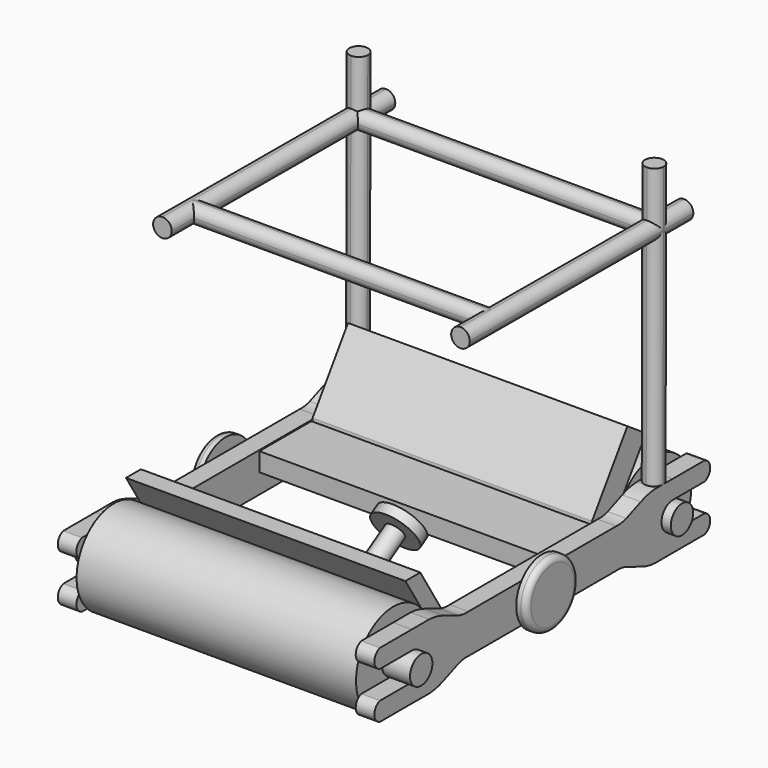
from build123d import *

# Parameters (mm, degrees)
F0_R           = 5
F1_DEPTH       = 30
F2_R           = 1.5
F3_DEPTH       = 3
F3_DEPTH_BACK  = 33
F5_DEPTH       = 2
F7_DEPTH       = 2
F8_R           = 3.5
F9_DEPTH       = 1.1
F10_R          = 0.6
F11_W          = 2
F11_H          = 2
F12_DEPTH      = 30
F13_W          = 2
F13_H          = 2
F14_DEPTH      = 25
F14_DEPTH_BACK = 5
F15_W          = 2
F15_H          = 1.9935706709
F16_DEPTH      = 31
F16_DEPTH_BACK = 1
F18_DEPTH      = 30
F19_R          = 1
F20_DEPTH      = 4.6
F21_R          = 2.5
F22_DEPTH      = 1.1
F23_R          = 0.99999
F24_R          = 0.99999
F25_R          = 0.99999
F26_R          = 0.99999
F27_T1_DEPTH   = 37
F28_T1_DEPTH   = 37
F29_R          = 3.5
F30_DEPTH      = 1.1
F31_R          = 0.6


# Not quite as in the source:
# - a fillet or chamfer that OpenCascade refuses, or shapes differently, is made with other operations: its cross-section is extruded or revolved along the edge and cut away or added
# - a fillet or chamfer is up to 0.001 mm smaller than in the source, because OpenCascade refuses the exact size


with BuildPart() as f1:
    # F0 (on Right) → F1 (new body)
    with BuildSketch(Plane.YZ):
        Circle(F0_R)
        with Locations((-35, 0)):
            Circle(F0_R)
    extrude(amount=F1_DEPTH)

    # F2 (on face) → F3 (join, two sides)
    with BuildSketch(Plane.YZ.offset(30)) as f3_sk:
        Circle(F2_R)
        with Locations((-35, 0)):
            Circle(F2_R)
    extrude(amount=F3_DEPTH)
    extrude(f3_sk.sketch, amount=-F3_DEPTH_BACK)


with BuildPart() as f5:
    # F4 (on face) → F5 (new body)
    with BuildSketch(Plane.YZ.offset(30)):
        with BuildLine():
            Line((-32.6922312379, 3.5074306652), (-35, 3.5))
            Line((-35, 3.5), (-39.2814344682, 3.5))
            ThreePointArc((-39.2814344682, 3.5), (-40.0388480928, 2.5), (-39.2814344682, 1.5))
            Line((-39.2814344682, 1.5), (-35, 1.5))
            ThreePointArc((-35, 1.5), (-33.9393398282, 1.0606601718), (-33.5, 0))
            ThreePointArc((-33.5, 0), (-33.9393398282, -1.0606601718), (-35, -1.5))
            Line((-35, -1.5), (-39.2814344682, -1.5))
            ThreePointArc((-39.2814344682, -1.5), (-40.0388480928, -2.5), (-39.2814344682, -3.5))
            Line((-39.2814344682, -3.5), (-35, -3.5))
            Line((-35, -3.5), (-32.6922312379, -3.5074306652))
            ThreePointArc((-32.6922312379, -3.5074306652), (-31.6914030649, -3.3770056429), (-30.7308007418, -3.0673108011))
            Line((-30.7308007418, -3.0673108011), (-28.7733972073, -2.2878439631))
            ThreePointArc((-28.7733972073, -2.2878439631), (-28.1066667518, -2.1263179414), (-27.4209757003, -2.1051533986))
            Line((-27.4209757003, -2.1051533986), (-17.5, -2.1051533986))
            Line((-17.5, -2.1051533986), (-7.5790242997, -2.1051533986))
            ThreePointArc((-7.5790242997, -2.1051533986), (-6.8933332482, -2.1263179414), (-6.2266027927, -2.2878439631))
            Line((-6.2266027927, -2.2878439631), (-4.2691992582, -3.0673108011))
            ThreePointArc((-4.2691992582, -3.0673108011), (-3.3085969351, -3.3770056429), (-2.3077687621, -3.5074306652))
            Line((-2.3077687621, -3.5074306652), (0, -3.5))
            Line((0, -3.5), (4.2814344682, -3.5))
            ThreePointArc((4.2814344682, -3.5), (5.0388480928, -2.5), (4.2814344682, -1.5))
            Line((4.2814344682, -1.5), (0, -1.5))
            ThreePointArc((0, -1.5), (-1.0606601718, -1.0606601718), (-1.5, 0))
            ThreePointArc((-1.5, 0), (-1.0606601718, 1.0606601718), (0, 1.5))
            Line((0, 1.5), (4.2814344682, 1.5))
            ThreePointArc((4.2814344682, 1.5), (5.0388480928, 2.5), (4.2814344682, 3.5))
            Line((4.2814344682, 3.5), (0, 3.5))
            Line((0, 3.5), (-2.3077687621, 3.5074306652))
            ThreePointArc((-2.3077687621, 3.5074306652), (-3.3085969351, 3.3770056429), (-4.2691992582, 3.0673108011))
            Line((-4.2691992582, 3.0673108011), (-6.2266027927, 2.2878439631))
            ThreePointArc((-6.2266027927, 2.2878439631), (-6.8933332482, 2.1263179414), (-7.5790242997, 2.1051533986))
            Line((-7.5790242997, 2.1051533986), (-17.5, 2.1051533986))
            Line((-17.5, 2.1051533986), (-27.4209757003, 2.1051533986))
            ThreePointArc((-27.4209757003, 2.1051533986), (-28.1066667518, 2.1263179414), (-28.7733972073, 2.2878439631))
            Line((-28.7733972073, 2.2878439631), (-30.7308007418, 3.0673108011))
            ThreePointArc((-30.7308007418, 3.0673108011), (-31.6914030649, 3.3770056429), (-32.6922312379, 3.5074306652))
        make_face()
    extrude(amount=F5_DEPTH)

    # F8 (on face) → F9 (join)
    with BuildSketch(Plane.YZ.offset(32)):
        with Locations((-17.5, 0)):
            Circle(F8_R)
    extrude(amount=F9_DEPTH)

    # F10
    f10_edges = [f5.edges().sort_by_distance(p)[0] for p in [
        (33.1, -21, 0),
    ]]
    fillet(f10_edges, radius=F10_R)


with BuildPart() as f7:
    # F6 (on face) → F7 (new body)
    with BuildSketch(Plane(origin=(0, 0, 0), x_dir=(0, -1, 0), z_dir=(-1, 0, 0))):
        with BuildLine():
            Line((2.2948030382, 3.5074306652), (-0.0129657239, 3.5))
            Line((-0.0129657239, 3.5), (-4.2944001921, 3.5))
            ThreePointArc((-4.2944001921, 3.5), (-5.0518138167, 2.5), (-4.2944001921, 1.5))
            Line((-4.2944001921, 1.5), (-0.0129657239, 1.5))
            ThreePointArc((-0.0129657239, 1.5), (1.0476944479, 1.0606601718), (1.4870342761, 0))
            ThreePointArc((1.4870342761, 0), (1.0476944479, -1.0606601718), (-0.0129657239, -1.5))
            Line((-0.0129657239, -1.5), (-4.2944001921, -1.5))
            ThreePointArc((-4.2944001921, -1.5), (-5.0518138167, -2.5), (-4.2944001921, -3.5))
            Line((-4.2944001921, -3.5), (-0.0129657239, -3.5))
            Line((-0.0129657239, -3.5), (2.2948030382, -3.5074306652))
            ThreePointArc((2.2948030382, -3.5074306652), (3.2956312112, -3.3770056429), (4.2562335343, -3.0673108011))
            Line((4.2562335343, -3.0673108011), (6.2136370689, -2.2878439631))
            ThreePointArc((6.2136370689, -2.2878439631), (6.8803675243, -2.1263179414), (7.5660585758, -2.1051533986))
            Line((7.5660585758, -2.1051533986), (17.4870342761, -2.1051533986))
            Line((17.4870342761, -2.1051533986), (27.4080099764, -2.1051533986))
            ThreePointArc((27.4080099764, -2.1051533986), (28.0937010279, -2.1263179414), (28.7604314834, -2.2878439631))
            Line((28.7604314834, -2.2878439631), (30.7178350179, -3.0673108011))
            ThreePointArc((30.7178350179, -3.0673108011), (31.6784373411, -3.3770056429), (32.679265514, -3.5074306652))
            Line((32.679265514, -3.5074306652), (34.9870342761, -3.5))
            Line((34.9870342761, -3.5), (39.2684687444, -3.5))
            ThreePointArc((39.2684687444, -3.5), (40.0258823689, -2.5), (39.2684687444, -1.5))
            Line((39.2684687444, -1.5), (34.9870342761, -1.5))
            ThreePointArc((34.9870342761, -1.5), (33.9263741043, -1.0606601718), (33.4870342761, 0))
            ThreePointArc((33.4870342761, 0), (33.9263741043, 1.0606601718), (34.9870342761, 1.5))
            Line((34.9870342761, 1.5), (39.2684687444, 1.5))
            ThreePointArc((39.2684687444, 1.5), (40.0258823689, 2.5), (39.2684687444, 3.5))
            Line((39.2684687444, 3.5), (34.9870342761, 3.5))
            Line((34.9870342761, 3.5), (32.679265514, 3.5074306652))
            ThreePointArc((32.679265514, 3.5074306652), (31.6784373411, 3.3770056429), (30.7178350179, 3.0673108011))
            Line((30.7178350179, 3.0673108011), (28.7604314834, 2.2878439631))
            ThreePointArc((28.7604314834, 2.2878439631), (28.0937010279, 2.1263179414), (27.4080099764, 2.1051533986))
            Line((27.4080099764, 2.1051533986), (17.4870342761, 2.1051533986))
            Line((17.4870342761, 2.1051533986), (7.5660585758, 2.1051533986))
            ThreePointArc((7.5660585758, 2.1051533986), (6.8803675243, 2.1263179414), (6.2136370689, 2.2878439631))
            Line((6.2136370689, 2.2878439631), (4.2562335343, 3.0673108011))
            ThreePointArc((4.2562335343, 3.0673108011), (3.2956312112, 3.3770056429), (2.2948030382, 3.5074306652))
        make_face()
    extrude(amount=F7_DEPTH)

    # F29 (on face) → F30 (join)
    with BuildSketch(Plane(origin=(-2, 0, 0), x_dir=(0, -1, 0), z_dir=(-1, 0, 0))):
        with Locations((17.5, 0)):
            Circle(F29_R)
    extrude(amount=F30_DEPTH)

    # F31
    f31_edges = [f7.edges().sort_by_distance(p)[0] for p in [
        (-3.1, -14, 0),
    ]]
    fillet(f31_edges, radius=F31_R)


with BuildPart() as f12:
    # F11 (on face) → F12 (new body)
    with BuildSketch(Plane(origin=(0, 0.011269352, 3.4999637144), x_dir=(1, 0, 0), z_dir=(0, 0.0032198316, 0.9999948163))):
        with Locations((31, -1.3190501353)):
            Rectangle(F11_W, F11_H)
        Polygon((-2.042085199, -1.9569919301), (-0.0425376123, -1.9995295424), (0, 1.80443e-05), (-1.9995475867, 0.0425556566), align=None)
    extrude(amount=F12_DEPTH)

    # F23 (radius 1 in the source; OpenCascade refuses exactly that, so slightly less here)
    f23_edges = [f12.edges().sort_by_distance(p)[0] for p in [
        (-2.042085, -1.897415, 18.506187),
        (-1.999548, 0.102122, 18.499749),
        (-0.042538, -1.939952, 18.506324),
        (0, 0.059585, 18.499886),
    ]]
    fillet(f23_edges, radius=F23_R)

    # F24 (radius 1 in the source; OpenCascade refuses exactly that, so slightly less here)
    f24_edges = [f12.edges().sort_by_distance(p)[0] for p in [
        (30, -0.259482, 18.500913),
        (32, -2.259471, 18.507353),
        (32, -0.259482, 18.500913),
        (30, -2.259471, 18.507353),
    ]]
    fillet(f24_edges, radius=F24_R)


with BuildPart() as f14:
    # F13 (on face) → F14 (new body, two sides)
    with BuildSketch(Plane(origin=(0, -2.3190381141, 0.0074669508), x_dir=(1, 0, 0), z_dir=(0, -0.9999948163, 0.0032198316))) as f14_sk:
        with Locations((31, 27.4999818572)):
            Rectangle(F13_W, F13_H)
        with Locations((-1, 27.4999818572)):
            Rectangle(F13_W, F13_H)
    extrude(amount=F14_DEPTH)
    extrude(f14_sk.sketch, amount=-F14_DEPTH_BACK)

    # F25 (radius 1 in the source; OpenCascade refuses exactly that, so slightly less here)
    f25_edges = [f14.edges().sort_by_distance(p)[0] for p in [
        (32, -12.227221, 28.539499),
        (32, -12.233661, 26.53951),
        (30, -12.227221, 28.539499),
        (30, -12.233661, 26.53951),
    ]]
    fillet(f25_edges, radius=F25_R)

    # F26 (radius 1 in the source; OpenCascade refuses exactly that, so slightly less here)
    f26_edges = [f14.edges().sort_by_distance(p)[0] for p in [
        (-2, -12.227221, 28.539499),
        (0, -12.227221, 28.539499),
        (-2, -12.233661, 26.53951),
        (0, -12.233661, 26.53951),
    ]]
    fillet(f26_edges, radius=F26_R)


with BuildPart() as f16:
    # F15 (on face) → F16 (new body, two sides)
    with BuildSketch(Plane(origin=(30, 0, 0), x_dir=(0, -1, 0), z_dir=(-1, 0, 0))) as f16_sk:
        with Locations((1.2272945373, 27.5040761109)):
            Rectangle(F15_W, F15_H)
        Polygon((24.226967344, 28.5781367507), (22.2270088133, 28.5652574912), (22.2398466702, 26.5717281563), (24.239805201, 26.5846074157), align=None)
    extrude(amount=F16_DEPTH)
    extrude(f16_sk.sketch, amount=-F16_DEPTH_BACK)

    # F27: fillet of radius 1 on 4 edges, made by hand

    # F27_s2 → F27_t1 (cut)
    with BuildSketch(Plane.YZ.offset(-3.5)):
        with BuildLine():
            ThreePointArc((-23.2269880787, 28.571697121), (-22.5217820829, 28.2742564693), (-22.233448443, 27.5652782259))
            Line((-22.233448443, 27.5652782259), (-22.2270088133, 28.5652574912))
            Line((-22.2270088133, 28.5652574912), (-23.2269880787, 28.571697121))
        make_face()
        with BuildLine():
            ThreePointArc((-23.2269880787, 28.571697121), (-23.9359663221, 28.283363481), (-24.2334069737, 27.5781574853))
            Line((-24.2334069737, 27.5781574853), (-24.226967344, 28.5781367507))
            Line((-24.226967344, 28.5781367507), (-23.2269880787, 28.571697121))
        make_face()
        with BuildLine():
            ThreePointArc((-23.2398259356, 26.578167786), (-22.5308476921, 26.8665014259), (-22.2334070405, 27.5717074217))
            Line((-22.2334070405, 27.5717074217), (-22.2398466702, 26.5717281563))
            Line((-22.2398466702, 26.5717281563), (-23.2398259356, 26.578167786))
        make_face()
        with BuildLine():
            ThreePointArc((-23.2398259356, 26.578167786), (-23.9450319313, 26.8756084376), (-24.2333655712, 27.5845866811))
            Line((-24.2333655712, 27.5845866811), (-24.239805201, 26.5846074157))
            Line((-24.239805201, 26.5846074157), (-23.2398259356, 26.578167786))
        make_face()
    extrude(amount=F27_T1_DEPTH, mode=Mode.SUBTRACT)

    # F28: fillet of radius 1 on 4 edges, made by hand

    # F28_s2 → F28_t1 (cut)
    with BuildSketch(Plane.YZ.offset(-3.5)):
        with BuildLine():
            ThreePointArc((-1.2272945373, 28.5008614464), (-0.5201877561, 28.2079682276), (-0.2272945373, 27.5008614464))
            Line((-0.2272945373, 27.5008614464), (-0.2272945373, 28.5008614464))
            Line((-0.2272945373, 28.5008614464), (-1.2272945373, 28.5008614464))
        make_face()
        with BuildLine():
            ThreePointArc((-1.2272945373, 28.5008614464), (-1.9344013185, 28.2079682276), (-2.2272945373, 27.5008614464))
            Line((-2.2272945373, 27.5008614464), (-2.2272945373, 28.5008614464))
            Line((-2.2272945373, 28.5008614464), (-1.2272945373, 28.5008614464))
        make_face()
        with BuildLine():
            ThreePointArc((-1.2272945373, 26.5072907755), (-0.5201877561, 26.8001839943), (-0.2272945373, 27.5072907755))
            Line((-0.2272945373, 27.5072907755), (-0.2272945373, 26.5072907755))
            Line((-0.2272945373, 26.5072907755), (-1.2272945373, 26.5072907755))
        make_face()
        with BuildLine():
            ThreePointArc((-1.2272945373, 26.5072907755), (-1.9344013185, 26.8001839943), (-2.2272945373, 27.5072907755))
            Line((-2.2272945373, 27.5072907755), (-2.2272945373, 26.5072907755))
            Line((-2.2272945373, 26.5072907755), (-1.2272945373, 26.5072907755))
        make_face()
    extrude(amount=F28_T1_DEPTH, mode=Mode.SUBTRACT)


with BuildPart() as f18:
    # F17 (on face) → F18 (new body)
    with BuildSketch(Plane.YZ):
        Polygon((-15.4621982947, 0), (-6.2136370689, 0), (-1.0889123601, 7.6042692763), (-3.5766951988, 9.2808540631), (-8.3262827247, 2.2332281806), (-8.4870342761, 1.1636078125), (-8.4870342761, 1.9946986687), (-15.4621982947, 1.9946986687), align=None)
        Polygon((-33.3720445633, 6.753959693), (-29.9563155987, 1.2678185567), (-27.9568070297, 1.2234847958), (-31.3720445633, 6.753959693), align=None)
    extrude(amount=F18_DEPTH)

    # F19 (on face) → F20 (join)
    with BuildSketch(Plane(origin=(0, -19.6918846162, -12.1603415076), x_dir=(-1, 0, 0), z_dir=(0, 0.8508422919, 0.525421159))):
        with Locations((-22.5, 18.2300905598)):
            Circle(F19_R)
    extrude(amount=F20_DEPTH)

    # F21 (on face) → F22 (join)
    with BuildSketch(Plane(origin=(0, -15.7780100736, -9.7434041761), x_dir=(-1, 0, 0), z_dir=(0, 0.8508422919, 0.525421159))):
        with Locations((-22.5, 18.2300905598)):
            Circle(F21_R)
    extrude(amount=F22_DEPTH)


solid = Compound([f1.part, f5.part, f7.part, f12.part, f14.part, f16.part, f18.part])
